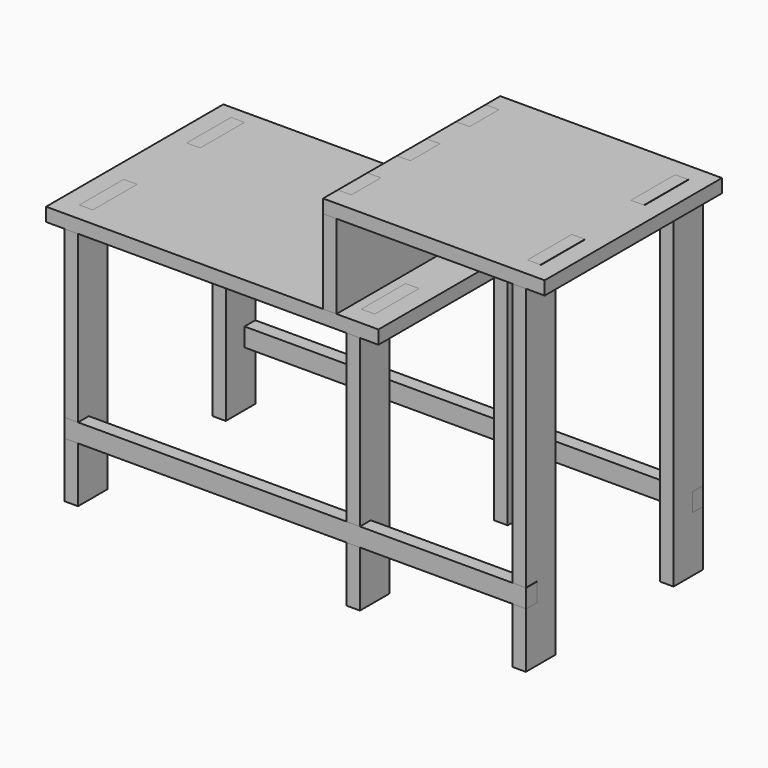
from build123d import *

# Parameters (mm, degrees)
F1_W      = 457.2
F1_H      = 304.8
F1_W_2    = 18.542
F1_H_2    = 76.2
F2_DEPTH  = 18.542
F4_W      = 18.542
F4_H      = 76.2
F5_DEPTH  = 18.542
F6_W      = 304.8
F6_H      = 152.4
F7_DEPTH  = 18.542
F11_DEPTH = 18.542
F18_DEPTH = 18.542
F24_DEPTH = 18.542
F27_W     = 635
F27_H     = 25.4
F28_DEPTH = 18.542
F29_W     = 635
F29_H     = 25.4
F30_DEPTH = 18.542


# Not quite as in the source:
# - a variable given as a bare number and used for a length is read in inches; the dataset says mm whatever the document's units were
# - a feature names something its author has since deleted; it is built from what else it names


with BuildPart() as f2:
    # F1 (on Top) → F2 (new body)
    with BuildSketch(Plane.XY):
        with Locations((-228.6, 152.4)):
            Rectangle(F1_W, F1_H)
        with Locations((-422.529, 63.5)):
            Rectangle(F1_W_2, F1_H_2, mode=Mode.SUBTRACT)
        with Locations((-34.671, 63.5)):
            Rectangle(F1_W_2, F1_H_2, mode=Mode.SUBTRACT)
        with Locations((-66.929, 88.9)):
            Rectangle(F1_W_2, F1_H_2, mode=Mode.SUBTRACT)
        with Locations((-422.529, 248.158)):
            Rectangle(F1_W_2, F1_H_2, mode=Mode.SUBTRACT)
        with Locations((-66.929, 215.9)):
            Rectangle(F1_W_2, F1_H_2, mode=Mode.SUBTRACT)
        with Locations((-34.671, 241.3)):
            Rectangle(F1_W_2, F1_H_2, mode=Mode.SUBTRACT)
    extrude(amount=F2_DEPTH)


with BuildPart() as f5:
    # F4 (on offset) → F5 (new body)
    with BuildSketch(Plane.XY.offset(152.4)):
        Polygon((-76.2, 25.4), (-76.2, 0), (228.6, 0), (228.6, 304.8), (-76.2, 304.8), (-76.2, 279.4), (-57.658, 279.4), (-57.658, 228.6), (-76.2, 228.6), (-76.2, 177.8), (-57.658, 177.8), (-57.658, 127), (-76.2, 127), (-76.2, 76.2), (-57.658, 76.2), (-57.658, 25.4), align=None)
        with Locations((193.929, 63.5)):
            Rectangle(F4_W, F4_H, mode=Mode.SUBTRACT)
        with Locations((193.929, 241.3)):
            Rectangle(F4_W, F4_H, mode=Mode.SUBTRACT)
    extrude(amount=-F5_DEPTH)


with BuildPart() as f7:
    # F6 (on face) → F7 (new body)
    with BuildSketch(Plane(origin=(-76.2, 0, 0), x_dir=(0, -1, 0), z_dir=(-1, 0, 0))):
        with Locations((-152.4, 76.2)):
            Rectangle(F6_W, F6_H)
    extrude(amount=-F7_DEPTH)

    # F8: cut F5
    add(f5.part, mode=Mode.SUBTRACT)

    # F16: cut F2
    add(f2.part, mode=Mode.SUBTRACT)


with BuildPart() as f11:
    # F10 (on Right) → F11 (new body)
    with BuildSketch(Plane.YZ):
        Polygon((127, 152.4), (0, 152.4), (0, -330.2), (50.8, -330.2), (50.8, 114.3), (127, 114.3), align=None)
    extrude(amount=F11_DEPTH)


with BuildPart() as f11b:
    # F10 (on Right) → F11, piece 2 (new body)
    with BuildSketch(Plane.YZ):
        Polygon((254, 114.3), (254, -330.2), (304.8, -330.2), (304.8, 152.4), (177.8, 152.4), (177.8, 114.3), align=None)
    extrude(amount=F11_DEPTH)


with BuildPart() as f11_1:
    # F12: moved
    add(f11.part.moved(Location((184.15, 0, 0))))

    # F13: cut F5
    add(f5.part, mode=Mode.SUBTRACT)


with BuildPart() as f11b_1:
    # F14: moved
    add(f11b.part.moved(Location((184.15, 0, 0))))

    # F15: cut F5
    add(f5.part, mode=Mode.SUBTRACT)


with BuildPart() as f18:
    # F17 (on Right) → F18 (new body)
    with BuildSketch(Plane.YZ):
        Polygon((127, 18.542), (0, 18.542), (0, -330.2), (50.8, -330.2), (50.8, -19.558), (127, -19.558), align=None)
    extrude(amount=-F18_DEPTH)


with BuildPart() as f18b:
    # F17 (on Right) → F18, piece 2 (new body)
    with BuildSketch(Plane.YZ):
        Polygon((304.8, 18.542), (177.8, 18.542), (177.8, -19.558), (254, -19.558), (254, -330.2), (304.8, -330.2), align=None)
    extrude(amount=-F18_DEPTH)


with BuildPart() as f18_1:
    # F19: moved
    add(f18.part.moved(Location((-25.4, 0, 0))))

    # F20: cut F2
    add(f2.part, mode=Mode.SUBTRACT)


with BuildPart() as f18b_1:
    # F21: moved
    add(f18b.part.moved(Location((-25.4, 0, 0))))

    # F22: cut F2
    add(f2.part, mode=Mode.SUBTRACT)


with BuildPart() as f24:
    # F23 (on face) → F24 (new body)
    with BuildSketch(Plane(origin=(-457.2, 0, 0), x_dir=(0, -1, 0), z_dir=(-1, 0, 0))):
        Polygon((-177.8, 18.542), (-304.8, 18.542), (-304.8, -329.946), (-254, -329.946), (-254, -18.796), (-177.8, -18.796), align=None)
    extrude(amount=-F24_DEPTH)


with BuildPart() as f24b:
    # F23 (on face) → F24, piece 2 (new body)
    with BuildSketch(Plane(origin=(-457.2, 0, 0), x_dir=(0, -1, 0), z_dir=(-1, 0, 0))):
        Polygon((-50.8, -18.796), (-50.8, -329.946), (0, -329.946), (0, 18.542), (-127, 18.542), (-127, -18.796), align=None)
    extrude(amount=-F24_DEPTH)


with BuildPart() as f24_1:
    # F25: moved
    add(f24.part.moved(Location((25.4, 0, 0))))

    # F26: cut F2
    add(f2.part, mode=Mode.SUBTRACT)


with BuildPart() as f24b_1:
    # F25: moved
    add(f24b.part.moved(Location((25.4, 0, 0))))

    # F26: cut F2
    add(f2.part, mode=Mode.SUBTRACT)


with BuildPart() as f28:
    # F27 (on face) → F28 (new body)
    with BuildSketch(Plane.XZ):
        with Locations((-114.3, -241.046)):
            Rectangle(F27_W, F27_H)
    extrude(amount=-F28_DEPTH)


with BuildPart() as f30:
    # F29 (on face) → F30 (new body)
    with BuildSketch(Plane(origin=(0, 304.8, 0), x_dir=(-1, 0, 0), z_dir=(0, 1, 0))):
        with Locations((114.808, -241.3)):
            Rectangle(F29_W, F29_H)
    extrude(amount=-F30_DEPTH)


with BuildPart() as f24b_2:
    add(f24b_1.part)

    # F31: cut F28
    add(f28.part, mode=Mode.SUBTRACT)


with BuildPart() as f18_2:
    add(f18_1.part)

    # F31: cut F28
    add(f28.part, mode=Mode.SUBTRACT)


with BuildPart() as f11_2:
    add(f11_1.part)

    # F31: cut F28
    add(f28.part, mode=Mode.SUBTRACT)


with BuildPart() as f11b_2:
    add(f11b_1.part)

    # F32: cut F30
    add(f30.part, mode=Mode.SUBTRACT)


with BuildPart() as f18b_2:
    add(f18b_1.part)

    # F32: cut F30
    add(f30.part, mode=Mode.SUBTRACT)


with BuildPart() as f24_2:
    add(f24_1.part)

    # F32: cut F30
    add(f30.part, mode=Mode.SUBTRACT)


solid = Compound([f2.part, f5.part, f7.part, f28.part, f30.part, f24b_2.part, f18_2.part, f11_2.part, f11b_2.part, f18b_2.part, f24_2.part])
